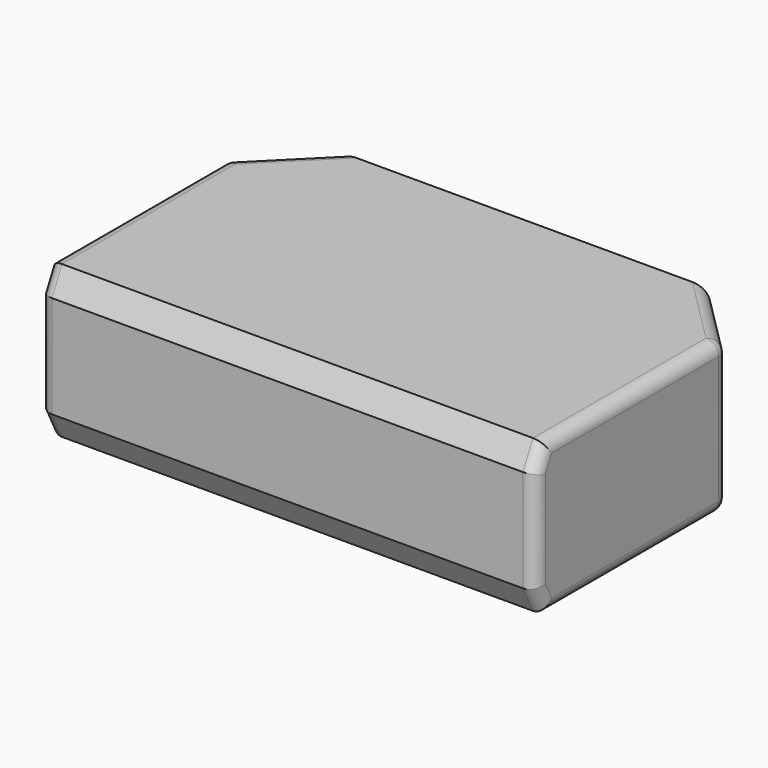
from build123d import *

# Parameters (mm, degrees)
F0_W         = 101.0383963585
F0_H         = 60.3721439838
F1_DEPTH     = 31.0119315982
F3_SIZE2     = 2.54
F3_SIZE      = 5.08
F4_SIZE      = 12.7
F5_R         = 2.54
F6_T1_DEPTH  = 23.2584097937
F6_T3_DEPTH  = 23.2584097937
F6_T5_DEPTH  = 25.9319315982
F6_T10_DEPTH = 2.54
F6_T16_DEPTH = 2.54
F6_T22_DEPTH = 2.54
F6_T28_DEPTH = 2.54


# Not quite as in the source:
# - a fillet or chamfer that OpenCascade refuses, or shapes differently, is made with other operations: its cross-section is extruded or revolved along the edge and cut away or added


with BuildPart() as f1:
    # F0 (on Top) → F1 (new body)
    with BuildSketch(Plane.XY):
        Rectangle(F0_W, F0_H)
    extrude(amount=F1_DEPTH)

    # F3
    f3_edges = [f1.edges().sort_by_distance(p)[0] for p in [
        (0, -30.186072, 31.011932),
        (0, -30.186072, 0),
    ]]
    f3_side = f1.faces().sort_by_distance((0, -30.186072, 15.505966))[0]
    chamfer(f3_edges, length=F3_SIZE, length2=F3_SIZE2, reference=f3_side)

    # F4
    f4_edges = [f1.edges().sort_by_distance(p)[0] for p in [
        (50.519198, 30.186072, 15.505966),
        (-50.519198, 30.186072, 15.505966),
    ]]
    chamfer(f4_edges, length=F4_SIZE)

    # F5
    f5_edges = [f1.edges().sort_by_distance(p)[0] for p in [
        (50.519198, -30.186072, 15.505966),
        (50.519198, -28.916072, 28.471932),
        (50.519198, -5.08, 31.011932),
        (50.519198, -5.08, 0),
        (50.519198, -28.916072, 2.54),
        (-50.519198, -5.08, 31.011932),
        (-50.519198, -30.186072, 15.505966),
        (-50.519198, -28.916072, 28.471932),
        (-50.519198, -28.916072, 2.54),
        (-50.519198, -5.08, 0),
    ]]
    fillet(f5_edges, radius=F5_R)

    # F6: fillet of radius 2.54 on 6 edges, made by hand

    # F6_s2 → F6_t1 (cut)
    with BuildSketch(Plane(origin=(15.7726143179, -15.7726143179, 0), x_dir=(0, 0, 1), z_dir=(-0.7071067812, 0.7071067812, 0))):
        with BuildLine():
            ThreePointArc((28.4719315982, 48.0869876945), (30.2679828224, 47.3430389187), (31.0119315982, 45.5469876945))
            Line((31.0119315982, 45.5469876945), (31.0119315982, 48.0869876945))
            Line((31.0119315982, 48.0869876945), (28.4719315982, 48.0869876945))
        make_face()
        with BuildLine():
            ThreePointArc((2.54, 48.0869876945), (0.7439487758, 47.3430389187), (0, 45.5469876945))
            Line((0, 45.5469876945), (0, 48.0869876945))
            Line((0, 48.0869876945), (2.54, 48.0869876945))
        make_face()
    extrude(amount=F6_T1_DEPTH, mode=Mode.SUBTRACT)

    # F6_s4 → F6_t3 (cut)
    with BuildSketch(Plane(origin=(0.6735649669, 0.6735649669, 0), x_dir=(0, 0, 1), z_dir=(-0.7071067812, -0.7071067812, 0))):
        with BuildLine():
            ThreePointArc((31.0119315982, 45.5469876945), (30.2679828224, 47.3430389187), (28.4719315982, 48.0869876945))
            Line((28.4719315982, 48.0869876945), (31.0119315982, 48.0869876945))
            Line((31.0119315982, 48.0869876945), (31.0119315982, 45.5469876945))
        make_face()
        with BuildLine():
            ThreePointArc((0, 45.5469876945), (0.7439487758, 47.3430389187), (2.54, 48.0869876945))
            Line((2.54, 48.0869876945), (0, 48.0869876945))
            Line((0, 48.0869876945), (0, 45.5469876945))
        make_face()
    extrude(amount=F6_T3_DEPTH, mode=Mode.SUBTRACT)

    # F6_s6 → F6_t5 (cut)
    with BuildSketch(Plane.XY.offset(2.54)):
        with BuildLine():
            ThreePointArc((50.5191981792, 16.4339695435), (50.3258521918, 17.4059854617), (49.7752494035, 18.2300207677))
            Line((49.7752494035, 18.2300207677), (50.5191981792, 17.4860719919))
            Line((50.5191981792, 17.4860719919), (50.5191981792, 16.4339695435))
        make_face()
        with BuildLine():
            ThreePointArc((-49.7752494035, 18.2300207677), (-50.3258521918, 17.4059854617), (-50.5191981792, 16.4339695435))
            Line((-50.5191981792, 16.4339695435), (-50.5191981792, 17.4860719919))
            Line((-50.5191981792, 17.4860719919), (-49.7752494035, 18.2300207677))
        make_face()
    extrude(amount=F6_T5_DEPTH, mode=Mode.SUBTRACT)


with BuildPart() as f6_tool8:
    # F6_s9 → F6_t10 (new body)
    with BuildSketch(Plane.XY.offset(2.54)):
        Polygon((-47.9791981792, 16.4339695435), (-50.5191981792, 16.4339695435), (-50.5191981792, 17.4860719919), (-49.7752494035, 18.2300207677), align=None)
    extrude(amount=-F6_T10_DEPTH)

    # F6_s11 → F6_t12 (revolve, cut)
    with BuildSketch(Plane(origin=(-47.9791981792, 16.4339695435, 2.54), x_dir=(0.9238795325, -0.3826834324, 0), z_dir=(0.3826834324, 0.9238795325, 0))):
        with BuildLine():
            ThreePointArc((0, -2.54), (2.54, 0), (0, 2.54))
            Line((0, 2.54), (0, -2.54))
        make_face()
    revolve(axis=Axis((-47.9791981792, 16.4339695435, 2.54), (0, 0, -1)), mode=Mode.SUBTRACT)


with BuildPart() as f1_1:
    add(f1.part)

    # F6_t7: cut F6_tool8
    add(f6_tool8.part, mode=Mode.SUBTRACT)


with BuildPart() as f6_tool14:
    # F6_s15 → F6_t16 (new body)
    with BuildSketch(Plane.XY.offset(28.4719315982)):
        Polygon((-47.9791981792, 16.4339695435), (-50.5191981792, 16.4339695435), (-50.5191981792, 17.4860719919), (-49.7752494035, 18.2300207677), align=None)
    extrude(amount=F6_T16_DEPTH)

    # F6_s17 → F6_t18 (revolve, cut)
    with BuildSketch(Plane(origin=(-47.9791981792, 16.4339695435, 28.4719315982), x_dir=(0.9238795325, -0.3826834324, 0), z_dir=(-0.3826834324, -0.9238795325, 0))):
        with BuildLine():
            ThreePointArc((0, -2.54), (2.54, 0), (0, 2.54))
            Line((0, 2.54), (0, -2.54))
        make_face()
    revolve(axis=Axis((-47.9791981792, 16.4339695435, 28.4719315982), (0, 0, 1)), mode=Mode.SUBTRACT)


with BuildPart() as f1_2:
    add(f1_1.part)

    # F6_t13: cut F6_tool14
    add(f6_tool14.part, mode=Mode.SUBTRACT)


with BuildPart() as f6_tool20:
    # F6_s21 → F6_t22 (new body)
    with BuildSketch(Plane.XY.offset(2.54)):
        Polygon((47.9791981792, 16.4339695435), (50.5191981792, 16.4339695435), (50.5191981792, 17.4860719919), (49.7752494035, 18.2300207677), align=None)
    extrude(amount=-F6_T22_DEPTH)

    # F6_s23 → F6_t24 (revolve, cut)
    with BuildSketch(Plane(origin=(47.9791981792, 16.4339695435, 2.54), x_dir=(-0.9238795325, -0.3826834324, 0), z_dir=(0.3826834324, -0.9238795325, 0))):
        with BuildLine():
            ThreePointArc((0, -2.54), (2.54, 0), (0, 2.54))
            Line((0, 2.54), (0, -2.54))
        make_face()
    revolve(axis=Axis((47.9791981792, 16.4339695435, 2.54), (0, 0, -1)), mode=Mode.SUBTRACT)


with BuildPart() as f1_3:
    add(f1_2.part)

    # F6_t19: cut F6_tool20
    add(f6_tool20.part, mode=Mode.SUBTRACT)


with BuildPart() as f6_tool26:
    # F6_s27 → F6_t28 (new body)
    with BuildSketch(Plane.XY.offset(28.4719315982)):
        Polygon((47.9791981792, 16.4339695435), (50.5191981792, 16.4339695435), (50.5191981792, 17.4860719919), (49.7752494035, 18.2300207677), align=None)
    extrude(amount=F6_T28_DEPTH)

    # F6_s29 → F6_t30 (revolve, cut)
    with BuildSketch(Plane(origin=(47.9791981792, 16.4339695435, 28.4719315982), x_dir=(-0.9238795325, -0.3826834324, 0), z_dir=(-0.3826834324, 0.9238795325, 0))):
        with BuildLine():
            ThreePointArc((0, -2.54), (2.54, 0), (0, 2.54))
            Line((0, 2.54), (0, -2.54))
        make_face()
    revolve(axis=Axis((47.9791981792, 16.4339695435, 28.4719315982), (0, 0, 1)), mode=Mode.SUBTRACT)


with BuildPart() as f1_4:
    add(f1_3.part)

    # F6_t25: cut F6_tool26
    add(f6_tool26.part, mode=Mode.SUBTRACT)


solid = f1_4.part
